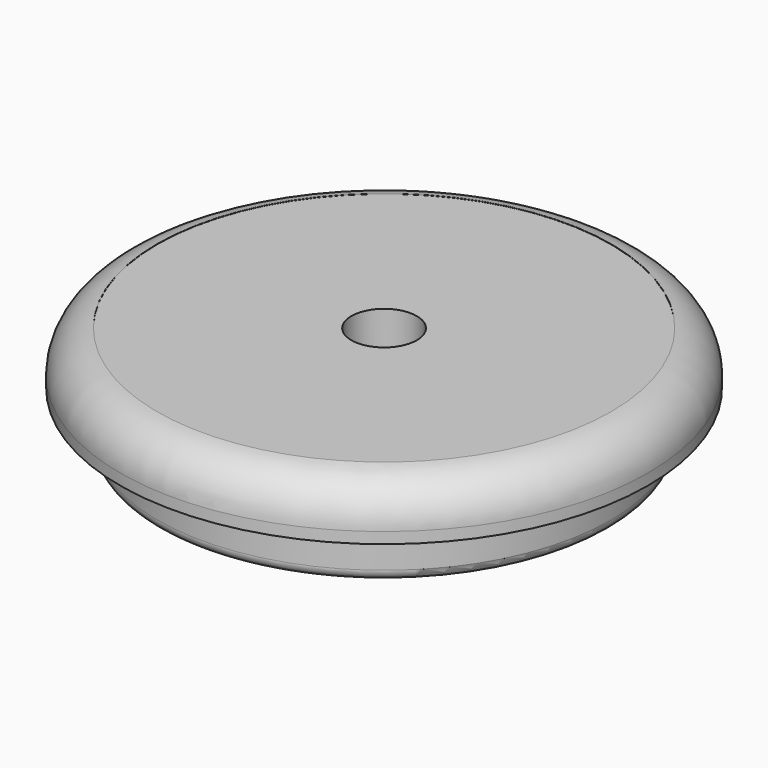
from build123d import *

# Parameters (mm, degrees)
F0_R     = 27.305
F1_DEPTH = 6.35
F2_R     = 3.937
F3_DEPTH = 12.7
F0_R_2   = 31.75
F4_DEPTH = 6.3754
F5_R     = 1.27


# Not quite as in the source:
# - a fillet or chamfer that OpenCascade refuses, or shapes differently, is made with other operations: its cross-section is extruded or revolved along the edge and cut away or added


with BuildPart() as f1:
    # F0 (on Top) → F1 (new body, symmetric)
    with BuildSketch(Plane.XY):
        Circle(F0_R)
    extrude(amount=F1_DEPTH, both=True)

    # F2 (on Top) → F3 (cut, symmetric)
    with BuildSketch(Plane.XY):
        Circle(F2_R)
    extrude(amount=F3_DEPTH, both=True, mode=Mode.SUBTRACT)

    # F0 (on Top) → F4 (join)
    with BuildSketch(Plane.XY):
        Circle(F0_R_2)
        Circle(F0_R, mode=Mode.SUBTRACT)
    extrude(amount=F4_DEPTH)

    # F5
    f5_edges = [f1.edges().sort_by_distance(p)[0] for p in [
        (-27.305, 0, -6.35),
    ]]
    fillet(f5_edges, radius=F5_R)

    # F6: fillet of radius 5.08 on 1 edges, made by hand

    # F6_s1 → F6_t2 (revolve, cut)
    with BuildSketch(Plane.XZ):
        with BuildLine():
            ThreePointArc((31.75, 1.3352437524), (30.48, 4.6953479175), (27.305, 6.3754))
            Line((27.305, 6.3754), (31.75, 6.3754))
            Line((31.75, 6.3754), (31.75, 1.3352437524))
        make_face()
    revolve(axis=Axis((0, 0, 6.3754), (0, 0, 1)), mode=Mode.SUBTRACT)


solid = f1.part
